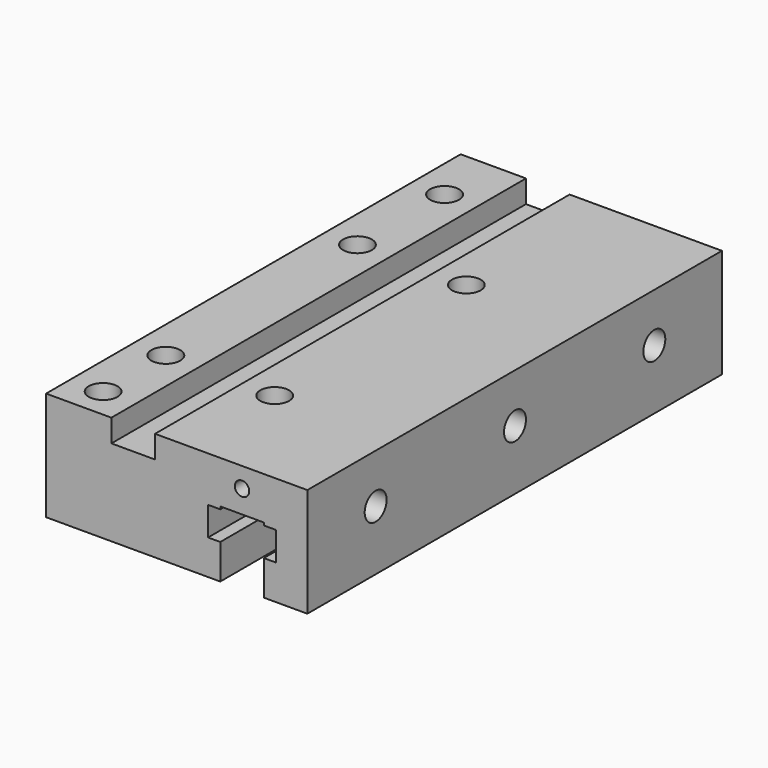
from build123d import *

# Parameters (mm, degrees)
F1_DEPTH = 75.565
F2_R     = 2.0955
F3_DEPTH = 13.97
F4_R     = 4
F5_DEPTH = 12.7
F6_R     = 4.2037
F7_DEPTH = 31.751


# Not quite as in the source:
# - a pattern or mirror of a feature is missing from the dataset's text; its kind, count and spacing are read off the source's solid


with BuildPart() as f1:
    # F0 (on Front) → F1 (new body, symmetric)
    with BuildSketch(Plane.XZ):
        Polygon((0, 31.75), (0, 0), (50.8, 0), (50.8, 10.16), (47.244, 10.16), (47.244, 18.542), (50.8, 18.542), (50.8, 19.304), (63.5, 19.304), (63.5, 18.542), (67.056, 18.542), (67.056, 10.16), (63.5, 10.16), (63.5, 0), (76.2, 0), (76.2, 31.75), (31.7754, 31.75), (31.7754, 25.146), (19.05, 25.146), (19.05, 31.75), align=None)
    extrude(amount=F1_DEPTH, both=True)

    # F2 (on face) → F3 (cut)
    with BuildSketch(Plane.XZ.offset(75.565)):
        with Locations((57.15, 25.9160771966)):
            Circle(F2_R)
    f3 = extrude(amount=-F3_DEPTH, mode=Mode.SUBTRACT)

    # F3_copies: F3 across plane
    add(f3.mirror(Plane.ZX), mode=Mode.SUBTRACT)

    # F4 (on face) → F5 (cut)
    with BuildSketch(Plane.YZ.offset(76.2)):
        with Locations((-50.673, 17.4752)):
            Circle(F4_R)
        with Locations((0.127, 17.4752)):
            Circle(F4_R)
        with Locations((50.927, 17.4752)):
            Circle(F4_R)
    extrude(amount=-F5_DEPTH, mode=Mode.SUBTRACT)

    # F6 (on face) → F7 (cut, through all)
    with BuildSketch(Plane.XY.offset(31.75)):
        with Locations((9.525, 57.785)):
            Circle(F6_R)
        with Locations((9.525, 26.035)):
            Circle(F6_R)
        with Locations((41.275, 26.035)):
            Circle(F6_R)
        with Locations((41.275, -43.815)):
            Circle(F6_R)
        with Locations((9.525, -43.815)):
            Circle(F6_R)
        with Locations((9.525, -66.675)):
            Circle(F6_R)
    extrude(amount=-F7_DEPTH, mode=Mode.SUBTRACT)


solid = f1.part
